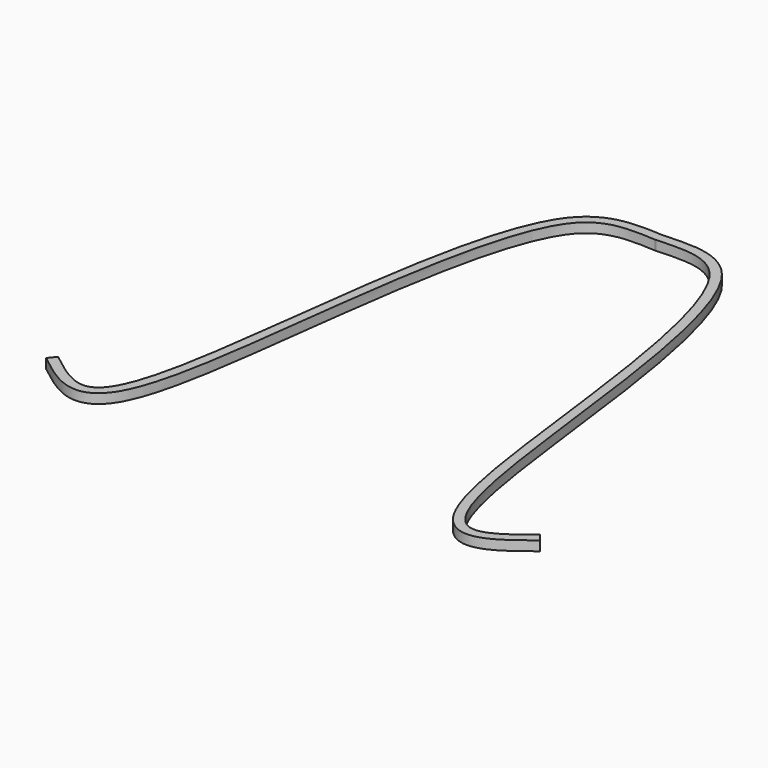
from build123d import *

# Parameters (mm, degrees)
F1_DEPTH = 2


# Not quite as in the source:
# - the dataset's text gives a spline's control points without its knots; the knots are read off the source's solid


with BuildPart() as f1:
    # F0 (on Top) → F1 (new body)
    with BuildSketch(Plane.XY):
        with BuildLine():
            add(Edge.make_bspline(
                [(-50.1542054117, 5.1819002256), (-46.4965038744, 2.3096156927), (-37.7342835737, -4.5710960294), (-29.2957694468, 22.0797782453), (-24.3990131261, 101.3615652653), (-5.9376875388, 100.3313473814), (0, 100)],
                knots=[0, 0, 0, 0, 0.1613209128, 0.386452903, 0.802665798, 1, 1, 1, 1], degree=3))
            Line((-50.1542054117, 5.1819002256), (-51.3894167035, 3.6089243629))
            add(Edge.make_bspline(
                [(-51.3894167035, 3.6089243629), (-50.6808714131, 3.0525247612), (-49.2457654062, 1.9252570157), (-47.0646979927, 0.3382478161), (-45.2237153327, -0.7795418417), (-43.7090954077, -1.4718673605), (-42.5370655831, -1.8625430901), (-41.3125297718, -2.0848884838), (-40.2462146545, -2.079681416), (-39.3828820846, -1.9249836914), (-38.5464659709, -1.6695897372), (-37.575450048, -1.1767625756), (-36.5585238956, -0.3681632238), (-35.3791515918, 0.9366588969), (-34.1593985328, 2.9370070061), (-32.9297764868, 5.9078848035), (-31.8540796356, 9.4635881522), (-30.8880785546, 13.6016753386), (-30.001738654, 18.3070171066), (-29.1708141346, 23.5682704795), (-28.3731911506, 29.3045368998), (-27.5865967966, 35.4046627257), (-26.5243982503, 43.8804538384), (-25.1194784391, 54.8417559352), (-23.4758218265, 65.5496877427), (-21.9401052545, 73.5088637389), (-20.6603463898, 79.0577925913), (-19.2376166083, 84.0664300619), (-17.9249545911, 87.6855562648), (-16.8014038945, 90.1812472495), (-15.9258288368, 91.8354096291), (-15.0234832002, 93.2556752804), (-14.1063559893, 94.4224474405), (-13.1626139631, 95.3765676268), (-11.8723098236, 96.4020458469), (-10.1844830645, 97.2955686748), (-7.9662938081, 97.9117713895), (-5.527332388, 98.167282181), (-2.8988838914, 98.158234508), (-1.0517317354, 98.0555792774), (-0.1114348496, 98.0031068445)],
                knots=[0, 0, 0, 0, 0.03125, 0.0625, 0.09375, 0.109375, 0.125, 0.140625, 0.15625, 0.1640625, 0.171875, 0.1875, 0.203125, 0.21875, 0.25, 0.28125, 0.3125, 0.34375, 0.375, 0.40625, 0.4375, 0.46875, 0.5, 0.5625, 0.625, 0.65625, 0.6875, 0.71875, 0.75, 0.765625, 0.78125, 0.796875, 0.8125, 0.828125, 0.84375, 0.875, 0.90625, 0.9375, 0.96875, 1, 1, 1, 1], degree=3))
            Line((-0.1114348496, 98.0031068445), (0.1114348496, 98.0031068445))
            add(Edge.make_bspline(
                [(51.3894167035, 3.6089243629), (50.6808714131, 3.0525247612), (49.2457654062, 1.9252570157), (47.0646979927, 0.3382478161), (45.2237153327, -0.7795418417), (43.7090954077, -1.4718673605), (42.5370655831, -1.8625430901), (41.3125297718, -2.0848884838), (40.2462146545, -2.079681416), (39.3828820846, -1.9249836914), (38.5464659709, -1.6695897372), (37.575450048, -1.1767625756), (36.5585238956, -0.3681632238), (35.3791515918, 0.9366588969), (34.1593985328, 2.9370070061), (32.9297764868, 5.9078848035), (31.8540796356, 9.4635881522), (30.8880785546, 13.6016753386), (30.001738654, 18.3070171066), (29.1708141346, 23.5682704795), (28.3731911506, 29.3045368998), (27.5865967966, 35.4046627257), (26.5243982503, 43.8804538384), (25.1194784391, 54.8417559352), (23.4758218265, 65.5496877427), (21.9401052545, 73.5088637389), (20.6603463898, 79.0577925913), (19.2376166083, 84.0664300619), (17.9249545911, 87.6855562648), (16.8014038945, 90.1812472495), (15.9258288368, 91.8354096291), (15.0234832002, 93.2556752804), (14.1063559893, 94.4224474405), (13.1626139631, 95.3765676268), (11.8723098236, 96.4020458469), (10.1844830645, 97.2955686748), (7.9662938081, 97.9117713895), (5.527332388, 98.167282181), (2.8988838914, 98.158234508), (1.0517317354, 98.0555792774), (0.1114348496, 98.0031068445)],
                knots=[0, 0, 0, 0, 0.03125, 0.0625, 0.09375, 0.109375, 0.125, 0.140625, 0.15625, 0.1640625, 0.171875, 0.1875, 0.203125, 0.21875, 0.25, 0.28125, 0.3125, 0.34375, 0.375, 0.40625, 0.4375, 0.46875, 0.5, 0.5625, 0.625, 0.65625, 0.6875, 0.71875, 0.75, 0.765625, 0.78125, 0.796875, 0.8125, 0.828125, 0.84375, 0.875, 0.90625, 0.9375, 0.96875, 1, 1, 1, 1], degree=3))
            Line((51.3894167035, 3.6089243629), (50.1542054117, 5.1819002256))
            add(Edge.make_bspline(
                [(50.1542054117, 5.1819002256), (46.4965038744, 2.3096156927), (37.7342835737, -4.5710960294), (29.2957694468, 22.0797782453), (24.3990131261, 101.3615652653), (5.9376875388, 100.3313473814), (0, 100)],
                knots=[0, 0, 0, 0, 0.1613209128, 0.386452903, 0.802665798, 1, 1, 1, 1], degree=3))
        make_face()
    extrude(amount=F1_DEPTH)


solid = f1.part
